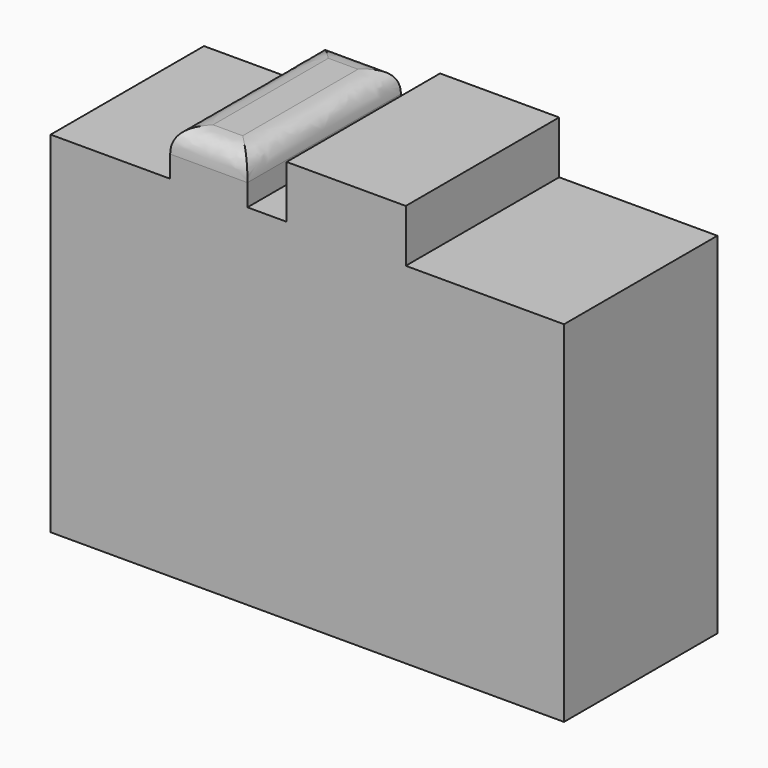
from build123d import *

# Parameters (mm, degrees)
F1_DEPTH     = 40.894
F2_T1_DEPTH  = 66.294
F2_T6_DEPTH  = 41.888453839
F2_T11_DEPTH = 41.888453839


# Not quite as in the source:
# - a fillet or chamfer that OpenCascade refuses, or shapes differently, is made with other operations: its cross-section is extruded or revolved along the edge and cut away or added


with BuildPart() as f1:
    # F0 (on Front) → F1 (new body)
    with BuildSketch(Plane.XZ):
        Polygon((-44.7658635676, 39.5274721086), (-44.7658635676, -35.146754235), (64.7440105677, -35.146754235), (64.7440105677, 39.5274721086), (30.9880006403, 39.5274721086), (30.9880006403, 50.7696404397), (5.5880006403, 50.7696404397), (5.5880006403, 39.5274721086), (-2.774850931, 39.5274721086), (-2.774850931, 49.2475219071), (-19.26330477, 49.2475219071), (-19.26330477, 39.5274721086), align=None)
    extrude(amount=F1_DEPTH)

    # F2: fillet of radius 5.08 on 4 edges, made by hand

    # F2_s2 → F2_t1 (cut)
    with BuildSketch(Plane.XZ.offset(-12.7)):
        with BuildLine():
            add(Edge.make_bspline(
                [(-2.774850931, 44.1675219071), (-2.774850931, 49.2475219071), (-7.854850931, 49.2475219071)],
                knots=[0, 0, 0, 1, 1, 1], degree=2, weights=[1, 1, 1]))
            Line((-7.854850931, 49.2475219071), (-2.774850931, 49.2475219071))
            Line((-2.774850931, 49.2475219071), (-2.774850931, 44.1675219071))
        make_face()
        with BuildLine():
            add(Edge.make_bspline(
                [(-14.18330477, 49.2475219071), (-19.26330477, 49.2475219071), (-19.26330477, 44.1675219071)],
                knots=[0, 0, 0, 1, 1, 1], degree=2, weights=[1, 1, 1]))
            Line((-19.26330477, 44.1675219071), (-19.26330477, 49.2475219071))
            Line((-19.26330477, 49.2475219071), (-14.18330477, 49.2475219071))
        make_face()
    extrude(amount=F2_T1_DEPTH, mode=Mode.SUBTRACT)


with BuildPart() as f2_tool4:
    # F2_s5 → F2_t6 (new body)
    with BuildSketch(Plane.YZ.offset(9.925149069)):
        with BuildLine():
            add(Edge.make_bspline(
                [(-5.08, 49.2475219071), (0, 49.2475219071), (0, 44.1675219071)],
                knots=[0, 0, 0, 1, 1, 1], degree=2, weights=[1, 1, 1]))
            Line((0, 44.1675219071), (0, 49.2475219071))
            Line((0, 49.2475219071), (-5.08, 49.2475219071))
        make_face()
    extrude(amount=-F2_T6_DEPTH)

    split(bisect_by=Plane.YZ.offset(5.5880006403), keep=Keep.BOTTOM)


with BuildPart() as f1_1:
    add(f1.part)

    # F2_t3: cut F2_tool4
    add(f2_tool4.part, mode=Mode.SUBTRACT)


with BuildPart() as f2_tool9:
    # F2_s10 → F2_t11 (new body)
    with BuildSketch(Plane.YZ.offset(9.925149069)):
        with BuildLine():
            add(Edge.make_bspline(
                [(-35.814, 49.2475219071), (-40.894, 49.2475219071), (-40.894, 44.1675219071)],
                knots=[0, 0, 0, 1, 1, 1], degree=2, weights=[1, 1, 1]))
            Line((-40.894, 44.1675219071), (-40.894, 49.2475219071))
            Line((-40.894, 49.2475219071), (-35.814, 49.2475219071))
        make_face()
    extrude(amount=-F2_T11_DEPTH)

    split(bisect_by=Plane.YZ.offset(5.5880006403), keep=Keep.BOTTOM)


with BuildPart() as f1_2:
    add(f1_1.part)

    # F2_t8: cut F2_tool9
    add(f2_tool9.part, mode=Mode.SUBTRACT)


solid = f1_2.part
